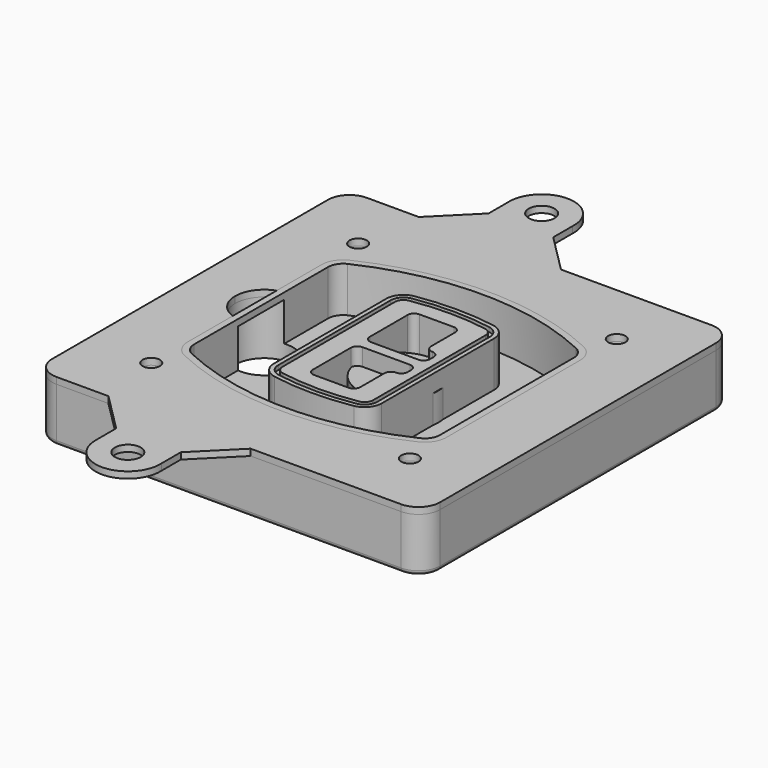
from build123d import *

# Parameters (mm, degrees)
F0_R      = 4
F1_DEPTH  = 25
F2_DEPTH  = 3
F3_DEPTH  = 18
F5_DEPTH  = 21
F6_DEPTH  = 2
F8_DEPTH  = 20
F9_DEPTH  = 16
F10_DEPTH = 25
F7_R      = 6
F7_R_2    = 4
F11_DEPTH = 6
F13_DEPTH = 9
F15_R     = 2
F16_R     = 6
F16_R_2   = 4
F17_DEPTH = 3


# Not quite as in the source:
# - a feature of the source that left no trace in its solid (it failed there, or was rolled back) is left out
# - a feature names something its author has since deleted; it is built from what else it names


with BuildPart() as f1:
    # F0 (on Top) → F1 (new body)
    with BuildSketch(Plane.XY):
        with BuildLine():
            ThreePointArc((-90, -80), (-87.0710678119, -87.0710678119), (-80, -90))
            Line((-80, -90), (80, -90))
            ThreePointArc((80, -90), (87.0710678119, -87.0710678119), (90, -80))
            Line((90, -80), (90, 80))
            ThreePointArc((90, 80), (87.0710678119, 87.0710678119), (80, 90))
            Line((80, 90), (-80, 90))
            ThreePointArc((-80, 90), (-87.0710678119, 87.0710678119), (-90, 80))
            Line((-90, 80), (-90, -80))
        make_face()
        with Locations((-60, -60)):
            Circle(F0_R, mode=Mode.SUBTRACT)
        with Locations((60, -60)):
            Circle(F0_R, mode=Mode.SUBTRACT)
        with Locations((-60, 60)):
            Circle(F0_R, mode=Mode.SUBTRACT)
        with BuildLine():
            ThreePointArc((-64, 38.8308515907), (-61.8195654598, 46.3340424013), (-55.9574468085, 51.5000594398))
            ThreePointArc((-55.9574468085, 51.5000594398), (0, 64), (55.9574468085, 51.5000594398))
            ThreePointArc((55.9574468085, 51.5000594398), (61.8195654598, 46.3340424013), (64, 38.8308515907))
            Line((64, 38.8308515907), (64, -38.8308515907))
            ThreePointArc((64, -38.8308515907), (61.8195654598, -46.3340424013), (55.9574468085, -51.5000594398))
            ThreePointArc((55.9574468085, -51.5000594398), (0, -64), (-55.9574468085, -51.5000594398))
            ThreePointArc((-55.9574468085, -51.5000594398), (-61.8195654598, -46.3340424013), (-64, -38.8308515907))
            Line((-64, -38.8308515907), (-64, 38.8308515907))
        make_face(mode=Mode.SUBTRACT)
        with Locations((60, 60)):
            Circle(F0_R, mode=Mode.SUBTRACT)
        with BuildLine():
            ThreePointArc((55.9574468085, 51.5000594398), (0, 64), (-55.9574468085, 51.5000594398))
            ThreePointArc((-55.9574468085, 51.5000594398), (-61.8195654598, 46.3340424013), (-64, 38.8308515907))
            Line((-64, 38.8308515907), (-64, -38.8308515907))
            ThreePointArc((-64, -38.8308515907), (-61.8195654598, -46.3340424013), (-55.9574468085, -51.5000594398))
            ThreePointArc((-55.9574468085, -51.5000594398), (0, -64), (55.9574468085, -51.5000594398))
            ThreePointArc((55.9574468085, -51.5000594398), (61.8195654598, -46.3340424013), (64, -38.8308515907))
            Line((64, -38.8308515907), (64, 38.8308515907))
            ThreePointArc((64, 38.8308515907), (61.8195654598, 46.3340424013), (55.9574468085, 51.5000594398))
        make_face()
        with BuildLine():
            Line((-60, -38.8308515907), (-60, 38.8308515907))
            ThreePointArc((-60, 38.8308515907), (-58.442546757, 44.1902735983), (-54.2553191489, 47.8802857686))
            ThreePointArc((-54.2553191489, 47.8802857686), (0, 60), (54.2553191489, 47.8802857686))
            ThreePointArc((54.2553191489, 47.8802857686), (58.442546757, 44.1902735983), (60, 38.8308515907))
            Line((60, 38.8308515907), (60, -38.8308515907))
            ThreePointArc((60, -38.8308515907), (58.442546757, -44.1902735983), (54.2553191489, -47.8802857686))
            ThreePointArc((54.2553191489, -47.8802857686), (0, -60), (-54.2553191489, -47.8802857686))
            ThreePointArc((-54.2553191489, -47.8802857686), (-58.442546757, -44.1902735983), (-60, -38.8308515907))
        make_face(mode=Mode.SUBTRACT)
        with BuildLine():
            ThreePointArc((-54.2553191489, 47.8802857686), (-58.442546757, 44.1902735983), (-60, 38.8308515907))
            Line((-60, 38.8308515907), (-60, -38.8308515907))
            ThreePointArc((-60, -38.8308515907), (-58.442546757, -44.1902735983), (-54.2553191489, -47.8802857686))
            ThreePointArc((-54.2553191489, -47.8802857686), (0, -60), (54.2553191489, -47.8802857686))
            ThreePointArc((54.2553191489, -47.8802857686), (58.442546757, -44.1902735983), (60, -38.8308515907))
            Line((60, -38.8308515907), (60, 38.8308515907))
            ThreePointArc((60, 38.8308515907), (58.442546757, 44.1902735983), (54.2553191489, 47.8802857686))
            ThreePointArc((54.2553191489, 47.8802857686), (0, 60), (-54.2553191489, 47.8802857686))
        make_face()
        with BuildLine():
            ThreePointArc((52.9787234043, 45.1654555152), (55.9097827299, 42.582446996), (57, 38.8308515907))
            Line((57, 38.8308515907), (57, -38.8308515907))
            ThreePointArc((57, -38.8308515907), (55.9097827299, -42.582446996), (52.9787234043, -45.1654555152))
            ThreePointArc((52.9787234043, -45.1654555152), (0, -57), (-52.9787234043, -45.1654555152))
            ThreePointArc((-52.9787234043, -45.1654555152), (-55.9097827299, -42.582446996), (-57, -38.8308515907))
            Line((-57, -38.8308515907), (-57, 38.8308515907))
            ThreePointArc((-57, 38.8308515907), (-55.9097827299, 42.582446996), (-52.9787234043, 45.1654555152))
            ThreePointArc((-52.9787234043, 45.1654555152), (0, 57), (52.9787234043, 45.1654555152))
        make_face(mode=Mode.SUBTRACT)
        with BuildLine():
            Line((57, -38.8308515907), (57, 38.8308515907))
            ThreePointArc((57, 38.8308515907), (55.9097827299, 42.582446996), (52.9787234043, 45.1654555152))
            ThreePointArc((52.9787234043, 45.1654555152), (0, 57), (-52.9787234043, 45.1654555152))
            ThreePointArc((-52.9787234043, 45.1654555152), (-55.9097827299, 42.582446996), (-57, 38.8308515907))
            Line((-57, 38.8308515907), (-57, -38.8308515907))
            ThreePointArc((-57, -38.8308515907), (-55.9097827299, -42.582446996), (-52.9787234043, -45.1654555152))
            ThreePointArc((-52.9787234043, -45.1654555152), (0, -57), (52.9787234043, -45.1654555152))
            ThreePointArc((52.9787234043, -45.1654555152), (55.9097827299, -42.582446996), (57, -38.8308515907))
        make_face()
    extrude(amount=-F1_DEPTH)

    # F0 (on Top) → F2 (join)
    with BuildSketch(Plane.XY):
        with BuildLine():
            ThreePointArc((-54.2553191489, 47.8802857686), (-58.442546757, 44.1902735983), (-60, 38.8308515907))
            Line((-60, 38.8308515907), (-60, -38.8308515907))
            ThreePointArc((-60, -38.8308515907), (-58.442546757, -44.1902735983), (-54.2553191489, -47.8802857686))
            ThreePointArc((-54.2553191489, -47.8802857686), (0, -60), (54.2553191489, -47.8802857686))
            ThreePointArc((54.2553191489, -47.8802857686), (58.442546757, -44.1902735983), (60, -38.8308515907))
            Line((60, -38.8308515907), (60, 38.8308515907))
            ThreePointArc((60, 38.8308515907), (58.442546757, 44.1902735983), (54.2553191489, 47.8802857686))
            ThreePointArc((54.2553191489, 47.8802857686), (0, 60), (-54.2553191489, 47.8802857686))
        make_face()
        with BuildLine():
            ThreePointArc((52.9787234043, 45.1654555152), (55.9097827299, 42.582446996), (57, 38.8308515907))
            Line((57, 38.8308515907), (57, -38.8308515907))
            ThreePointArc((57, -38.8308515907), (55.9097827299, -42.582446996), (52.9787234043, -45.1654555152))
            ThreePointArc((52.9787234043, -45.1654555152), (0, -57), (-52.9787234043, -45.1654555152))
            ThreePointArc((-52.9787234043, -45.1654555152), (-55.9097827299, -42.582446996), (-57, -38.8308515907))
            Line((-57, -38.8308515907), (-57, 38.8308515907))
            ThreePointArc((-57, 38.8308515907), (-55.9097827299, 42.582446996), (-52.9787234043, 45.1654555152))
            ThreePointArc((-52.9787234043, 45.1654555152), (0, 57), (52.9787234043, 45.1654555152))
        make_face(mode=Mode.SUBTRACT)
    extrude(amount=F2_DEPTH)

    # F0 (on Top) → F3 (cut)
    with BuildSketch(Plane.XY):
        with BuildLine():
            Line((57, -38.8308515907), (57, 38.8308515907))
            ThreePointArc((57, 38.8308515907), (55.9097827299, 42.582446996), (52.9787234043, 45.1654555152))
            ThreePointArc((52.9787234043, 45.1654555152), (0, 57), (-52.9787234043, 45.1654555152))
            ThreePointArc((-52.9787234043, 45.1654555152), (-55.9097827299, 42.582446996), (-57, 38.8308515907))
            Line((-57, 38.8308515907), (-57, -38.8308515907))
            ThreePointArc((-57, -38.8308515907), (-55.9097827299, -42.582446996), (-52.9787234043, -45.1654555152))
            ThreePointArc((-52.9787234043, -45.1654555152), (0, -57), (52.9787234043, -45.1654555152))
            ThreePointArc((52.9787234043, -45.1654555152), (55.9097827299, -42.582446996), (57, -38.8308515907))
        make_face()
    extrude(amount=-F3_DEPTH, mode=Mode.SUBTRACT)

    # F4 (on face) → F5 (join, through all)
    with BuildSketch(Plane.XY.offset(3)):
        with BuildLine():
            ThreePointArc((-25, -32.5662280692), (-23.1122504785, -37.7276614059), (-18.3399014778, -40.4532214146))
            ThreePointArc((-18.3399014778, -40.4532214146), (0, -42), (18.3399014778, -40.4532214146))
            ThreePointArc((18.3399014778, -40.4532214146), (23.1122504785, -37.7276614059), (25, -32.5662280692))
            Line((25, -32.5662280692), (25, 32.5662280692))
            ThreePointArc((25, 32.5662280692), (23.1122504785, 37.7276614059), (18.3399014778, 40.4532214146))
            ThreePointArc((18.3399014778, 40.4532214146), (0, 42), (-18.3399014778, 40.4532214146))
            ThreePointArc((-18.3399014778, 40.4532214146), (-23.1122504785, 37.7276614059), (-25, 32.5662280692))
            Line((-25, 32.5662280692), (-25, -32.5662280692))
        make_face()
        with BuildLine():
            ThreePointArc((18.0049261084, 38.4814730782), (21.5841878588, 36.4373030717), (23, 32.5662280692))
            Line((23, 32.5662280692), (23, -32.5662280692))
            ThreePointArc((23, -32.5662280692), (21.5841878588, -36.4373030717), (18.0049261084, -38.4814730782))
            ThreePointArc((18.0049261084, -38.4814730782), (0, -40), (-18.0049261084, -38.4814730782))
            ThreePointArc((-18.0049261084, -38.4814730782), (-21.5841878588, -36.4373030717), (-23, -32.5662280692))
            Line((-23, -32.5662280692), (-23, 32.5662280692))
            ThreePointArc((-23, 32.5662280692), (-21.5841878588, 36.4373030717), (-18.0049261084, 38.4814730782))
            ThreePointArc((-18.0049261084, 38.4814730782), (0, 40), (18.0049261084, 38.4814730782))
        make_face(mode=Mode.SUBTRACT)
        with BuildLine():
            Line((23, -32.5662280692), (23, 32.5662280692))
            ThreePointArc((23, 32.5662280692), (21.5841878588, 36.4373030717), (18.0049261084, 38.4814730782))
            ThreePointArc((18.0049261084, 38.4814730782), (0, 40), (-18.0049261084, 38.4814730782))
            ThreePointArc((-18.0049261084, 38.4814730782), (-21.5841878588, 36.4373030717), (-23, 32.5662280692))
            Line((-23, 32.5662280692), (-23, -32.5662280692))
            ThreePointArc((-23, -32.5662280692), (-21.5841878588, -36.4373030717), (-18.0049261084, -38.4814730782))
            ThreePointArc((-18.0049261084, -38.4814730782), (0, -40), (18.0049261084, -38.4814730782))
            ThreePointArc((18.0049261084, -38.4814730782), (21.5841878588, -36.4373030717), (23, -32.5662280692))
        make_face()
        with BuildLine():
            ThreePointArc((17.6699507389, 36.5097247419), (20.0561252392, 35.1469447375), (21, 32.5662280692))
            Line((21, 32.5662280692), (21, -32.5662280692))
            ThreePointArc((21, -32.5662280692), (20.0561252392, -35.1469447375), (17.6699507389, -36.5097247419))
            ThreePointArc((17.6699507389, -36.5097247419), (0, -38), (-17.6699507389, -36.5097247419))
            ThreePointArc((-17.6699507389, -36.5097247419), (-20.0561252392, -35.1469447375), (-21, -32.5662280692))
            Line((-21, -32.5662280692), (-21, 32.5662280692))
            ThreePointArc((-21, 32.5662280692), (-20.0561252392, 35.1469447375), (-17.6699507389, 36.5097247419))
            ThreePointArc((-17.6699507389, 36.5097247419), (0, 38), (17.6699507389, 36.5097247419))
        make_face(mode=Mode.SUBTRACT)
        with BuildLine():
            Line((21, -32.5662280692), (21, 32.5662280692))
            ThreePointArc((21, 32.5662280692), (20.0561252392, 35.1469447375), (17.6699507389, 36.5097247419))
            ThreePointArc((17.6699507389, 36.5097247419), (0, 38), (-17.6699507389, 36.5097247419))
            ThreePointArc((-17.6699507389, 36.5097247419), (-20.0561252392, 35.1469447375), (-21, 32.5662280692))
            Line((-21, 32.5662280692), (-21, -32.5662280692))
            ThreePointArc((-21, -32.5662280692), (-20.0561252392, -35.1469447375), (-17.6699507389, -36.5097247419))
            ThreePointArc((-17.6699507389, -36.5097247419), (0, -38), (17.6699507389, -36.5097247419))
            ThreePointArc((17.6699507389, -36.5097247419), (20.0561252392, -35.1469447375), (21, -32.5662280692))
        make_face()
        with BuildLine():
            Line((-8, -2.5), (14, -2.5))
            ThreePointArc((14, -2.5), (16.1213203436, -3.3786796564), (17, -5.5))
            Line((17, -5.5), (17, -7.5))
            ThreePointArc((17, -7.5), (16.1213203436, -9.6213203436), (14, -10.5))
            ThreePointArc((14, -10.5), (11.8786796564, -11.3786796564), (11, -13.5))
            Line((11, -13.5), (11, -27.5))
            ThreePointArc((11, -27.5), (10.1213203436, -29.6213203436), (8, -30.5))
            Line((8, -30.5), (-8, -30.5))
            ThreePointArc((-8, -30.5), (-10.1213203436, -29.6213203436), (-11, -27.5))
            Line((-11, -27.5), (-11, -5.5))
            ThreePointArc((-11, -5.5), (-10.1213203436, -3.3786796564), (-8, -2.5))
        make_face(mode=Mode.SUBTRACT)
        with BuildLine():
            ThreePointArc((-8, 2.5), (-10.1213203436, 3.3786796564), (-11, 5.5))
            Line((-11, 5.5), (-11, 27.5))
            ThreePointArc((-11, 27.5), (-10.1213203436, 29.6213203436), (-8, 30.5))
            Line((-8, 30.5), (8, 30.5))
            ThreePointArc((8, 30.5), (10.1213203436, 29.6213203436), (11, 27.5))
            Line((11, 27.5), (11, 13.5))
            ThreePointArc((11, 13.5), (11.8786796564, 11.3786796564), (14, 10.5))
            ThreePointArc((14, 10.5), (16.1213203436, 9.6213203436), (17, 7.5))
            Line((17, 7.5), (17, 5.5))
            ThreePointArc((17, 5.5), (16.1213203436, 3.3786796564), (14, 2.5))
            Line((14, 2.5), (-8, 2.5))
        make_face(mode=Mode.SUBTRACT)
    extrude(amount=-F5_DEPTH)

    # F4 (on face) → F6 (cut)
    with BuildSketch(Plane.XY.offset(3)):
        with BuildLine():
            Line((23, -32.5662280692), (23, 32.5662280692))
            ThreePointArc((23, 32.5662280692), (21.5841878588, 36.4373030717), (18.0049261084, 38.4814730782))
            ThreePointArc((18.0049261084, 38.4814730782), (0, 40), (-18.0049261084, 38.4814730782))
            ThreePointArc((-18.0049261084, 38.4814730782), (-21.5841878588, 36.4373030717), (-23, 32.5662280692))
            Line((-23, 32.5662280692), (-23, -32.5662280692))
            ThreePointArc((-23, -32.5662280692), (-21.5841878588, -36.4373030717), (-18.0049261084, -38.4814730782))
            ThreePointArc((-18.0049261084, -38.4814730782), (0, -40), (18.0049261084, -38.4814730782))
            ThreePointArc((18.0049261084, -38.4814730782), (21.5841878588, -36.4373030717), (23, -32.5662280692))
        make_face()
        with BuildLine():
            ThreePointArc((17.6699507389, 36.5097247419), (20.0561252392, 35.1469447375), (21, 32.5662280692))
            Line((21, 32.5662280692), (21, -32.5662280692))
            ThreePointArc((21, -32.5662280692), (20.0561252392, -35.1469447375), (17.6699507389, -36.5097247419))
            ThreePointArc((17.6699507389, -36.5097247419), (0, -38), (-17.6699507389, -36.5097247419))
            ThreePointArc((-17.6699507389, -36.5097247419), (-20.0561252392, -35.1469447375), (-21, -32.5662280692))
            Line((-21, -32.5662280692), (-21, 32.5662280692))
            ThreePointArc((-21, 32.5662280692), (-20.0561252392, 35.1469447375), (-17.6699507389, 36.5097247419))
            ThreePointArc((-17.6699507389, 36.5097247419), (0, 38), (17.6699507389, 36.5097247419))
        make_face(mode=Mode.SUBTRACT)
    extrude(amount=-F6_DEPTH, mode=Mode.SUBTRACT)

    # F7 (on face) → F8 (join)
    with BuildSketch(Plane(origin=(0, 0, -25), x_dir=(1, 0, 0), z_dir=(0, 0, -1))):
        with BuildLine():
            ThreePointArc((-6.71157564, 0), (6.7567035675, 13.4682792075), (20.224982775, 0))
            Line((20.224982775, 0), (25.224982775, 0))
            ThreePointArc((25.224982775, 0), (6.7567035675, 18.4682792075), (-11.71157564, 0))
            Line((-11.71157564, 0), (-6.71157564, 0))
        make_face()
        with BuildLine():
            Line((-6.71157564, 0), (20.224982775, 0))
            ThreePointArc((20.224982775, 0), (6.7567035675, 13.4682792075), (-6.71157564, 0))
        make_face()
        with BuildLine():
            ThreePointArc((-6.71157564, 0), (6.7567035675, -13.4682792075), (20.224982775, 0))
            Line((20.224982775, 0), (-6.71157564, 0))
        make_face()
        with BuildLine():
            Line((25.224982775, 0), (20.224982775, 0))
            ThreePointArc((20.224982775, 0), (6.7567035675, -13.4682792075), (-6.71157564, 0))
            Line((-6.71157564, 0), (-11.71157564, 0))
            ThreePointArc((-11.71157564, 0), (6.7567035675, -18.4682792075), (25.224982775, 0))
        make_face()
    extrude(amount=-F8_DEPTH)

    # F7 (on face) → F9 (cut)
    with BuildSketch(Plane(origin=(0, 0, -25), x_dir=(1, 0, 0), z_dir=(0, 0, -1))):
        with BuildLine():
            Line((-6.71157564, 0), (20.224982775, 0))
            ThreePointArc((20.224982775, 0), (6.7567035675, 13.4682792075), (-6.71157564, 0))
        make_face()
        with BuildLine():
            ThreePointArc((-6.71157564, 0), (6.7567035675, -13.4682792075), (20.224982775, 0))
            Line((20.224982775, 0), (-6.71157564, 0))
        make_face()
    extrude(amount=-F9_DEPTH, mode=Mode.SUBTRACT)

    # F7 (on face) → F10 (cut)
    with BuildSketch(Plane(origin=(0, 0, -25), x_dir=(1, 0, 0), z_dir=(0, 0, -1))):
        with BuildLine():
            Line((-69.0318229325, 0), (-42.0952645175, 0))
            ThreePointArc((-42.0952645175, 0), (-55.563543725, 13.4682792075), (-69.0318229325, 0))
        make_face()
        with BuildLine():
            ThreePointArc((-69.0318229325, 0), (-55.563543725, -13.4682792075), (-42.0952645175, 0))
            Line((-42.0952645175, 0), (-69.0318229325, 0))
        make_face()
    extrude(amount=-F10_DEPTH, mode=Mode.SUBTRACT)

    # F7 (on face) → F11 (cut)
    with BuildSketch(Plane(origin=(0, 0, -25), x_dir=(1, 0, 0), z_dir=(0, 0, -1))):
        with Locations((60, -60)):
            Circle(F7_R)
        with Locations((60, -60)):
            Circle(F7_R_2, mode=Mode.SUBTRACT)
        with Locations((-60, -60)):
            Circle(F7_R)
        with Locations((-60, -60)):
            Circle(F7_R_2, mode=Mode.SUBTRACT)
        with Locations((-60, 60)):
            Circle(F7_R)
        with Locations((-60, 60)):
            Circle(F7_R_2, mode=Mode.SUBTRACT)
        with Locations((60, 60)):
            Circle(F7_R)
        with Locations((60, 60)):
            Circle(F7_R_2, mode=Mode.SUBTRACT)
    extrude(amount=-F11_DEPTH, mode=Mode.SUBTRACT)

    # F12 (on face) → F13 (cut, through all)
    with BuildSketch(Plane(origin=(0, 0, -9), x_dir=(1, 0, 0), z_dir=(0, 0, -1))):
        with BuildLine():
            ThreePointArc((20.224982775, 0), (20.1663399806, 1.2554664788), (19.9909222755, 2.5))
            Line((19.9909222755, 2.5), (14, 2.5))
            ThreePointArc((14, 2.5), (16.1213203436, 3.3786796564), (17, 5.5))
            Line((17, 5.5), (17, 7.5))
            ThreePointArc((17, 7.5), (16.1213203436, 9.6213203436), (14, 10.5))
            ThreePointArc((14, 10.5), (12.1627255951, 11.1284134507), (11.0951631559, 12.750384826))
            ThreePointArc((11.0951631559, 12.750384826), (11.0476113807, 12.7664660322), (11, 12.7823698976))
            Line((11, 12.7823698976), (11, -12.7823698976))
            ThreePointArc((11, -12.7823698976), (11.0476113807, -12.7664660322), (11.0951631559, -12.750384826))
            ThreePointArc((11.0951631559, -12.750384826), (12.1627255951, -11.1284134507), (14, -10.5))
            ThreePointArc((14, -10.5), (16.1213203436, -9.6213203436), (17, -7.5))
            Line((17, -7.5), (17, -5.5))
            ThreePointArc((17, -5.5), (16.1213203436, -3.3786796564), (14, -2.5))
            Line((14, -2.5), (19.9909222755, -2.5))
            ThreePointArc((19.9909222755, -2.5), (20.1663399806, -1.2554664788), (20.224982775, 0))
        make_face()
    extrude(amount=F13_DEPTH, mode=Mode.SUBTRACT)

    # F15
    f15_edges = [f1.edges().sort_by_distance(p)[0] for p in [
        (0, -90, -25),
        (-87.071068, -87.071068, -25),
        (-90, 0, -25),
        (-87.071068, 87.071068, -25),
        (87.071068, -87.071068, -25),
        (0, 90, -25),
        (90, 0, -25),
        (87.071068, 87.071068, -25),
    ]]
    fillet(f15_edges, radius=F15_R)


with BuildPart() as f17:
    # F16 (on face) → F17 (new body, through all)
    with BuildSketch(Plane.XY):
        with BuildLine():
            Line((10.1193234926, -90), (-55.8578643763, -90))
            Line((-55.8578643763, -90), (-37.8578643763, -108))
            Line((-37.8578643763, -108), (-37.8578643763, -120))
            ThreePointArc((-37.8578643763, -120), (-22.4442329176, -134.9942958826), (-7.8806765074, -119.1730516697))
            Line((-7.8806765074, -119.1730516697), (-7.8806765074, -108))
            Line((-7.8806765074, -108), (10.1193234926, -90))
        make_face()
        with Locations((-22.8578643763, -120)):
            Circle(F16_R, mode=Mode.SUBTRACT)
        with BuildLine():
            Line((-37.8578643763, 108), (-55.8578643763, 90))
            Line((-55.8578643763, 90), (10.1193234926, 90))
            Line((10.1193234926, 90), (-7.8806765074, 108))
            Line((-7.8806765074, 108), (-7.8806765074, 119.1730516697))
            ThreePointArc((-7.8806765074, 119.1730516697), (-22.4442329176, 134.9942958826), (-37.8578643763, 120))
            Line((-37.8578643763, 120), (-37.8578643763, 108))
        make_face()
        with Locations((-22.8578643763, 120)):
            Circle(F16_R, mode=Mode.SUBTRACT)
        with BuildLine():
            Line((10.1193234926, 90), (-55.8578643763, 90))
            Line((-55.8578643763, 90), (-80, 90))
            ThreePointArc((-80, 90), (-87.0710678119, 87.0710678119), (-90, 80))
            Line((-90, 80), (-90, -80))
            ThreePointArc((-90, -80), (-87.0710678119, -87.0710678119), (-80, -90))
            Line((-80, -90), (-55.8578643763, -90))
            Line((-55.8578643763, -90), (10.1193234926, -90))
            Line((10.1193234926, -90), (80, -90))
            ThreePointArc((80, -90), (87.0710678119, -87.0710678119), (90, -80))
            Line((90, -80), (90, 80))
            ThreePointArc((90, 80), (87.0710678119, 87.0710678119), (80, 90))
            Line((80, 90), (10.1193234926, 90))
        make_face()
        with Locations((-60, -60)):
            Circle(F16_R_2, mode=Mode.SUBTRACT)
        with Locations((60, -60)):
            Circle(F16_R_2, mode=Mode.SUBTRACT)
        with BuildLine():
            ThreePointArc((-60, 38.8308515907), (-58.442546757, 44.1902735983), (-54.2553191489, 47.8802857686))
            ThreePointArc((-54.2553191489, 47.8802857686), (0, 60), (54.2553191489, 47.8802857686))
            ThreePointArc((54.2553191489, 47.8802857686), (58.442546757, 44.1902735983), (60, 38.8308515907))
            Line((60, 38.8308515907), (60, -38.8308515907))
            ThreePointArc((60, -38.8308515907), (58.442546757, -44.1902735983), (54.2553191489, -47.8802857686))
            ThreePointArc((54.2553191489, -47.8802857686), (0, -60), (-54.2553191489, -47.8802857686))
            ThreePointArc((-54.2553191489, -47.8802857686), (-58.442546757, -44.1902735983), (-60, -38.8308515907))
            Line((-60, -38.8308515907), (-60, -12.7166190685))
            ThreePointArc((-60, -12.7166190685), (-66.5441169481, -7.798817635), (-69.0318229325, 0))
            ThreePointArc((-69.0318229325, 0), (-66.5441169481, 7.798817635), (-60, 12.7166190685))
            Line((-60, 12.7166190685), (-60, 38.8308515907))
        make_face(mode=Mode.SUBTRACT)
        with Locations((-60, 60)):
            Circle(F16_R_2, mode=Mode.SUBTRACT)
        with Locations((60, 60)):
            Circle(F16_R_2, mode=Mode.SUBTRACT)
    extrude(amount=F17_DEPTH)


solid = Compound([f1.part, f17.part])
